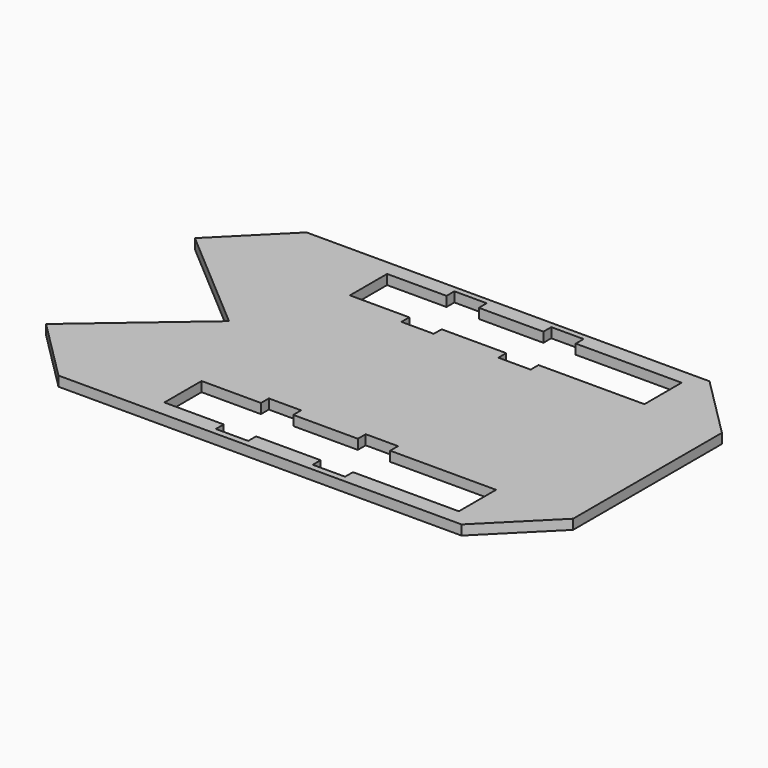
from build123d import *

# Parameters (mm, degrees)
F1_DEPTH = 3.175


# Not quite as in the source:
# - a length typed as a fraction of an inch, garbled in the dataset ("3 / 203.2 mm" for 3/8 in), is restored


with BuildPart() as f1:
    # F0 (on Top) → F1 (new body)
    with BuildSketch(Plane.XY):
        Polygon((84.4656275958, 81.8700266516), (-45.5343724042, 81.8700266516), (-65.5343724042, 61.8700266516), (-30.5343724042, 31.8700266516), (-65.5343724042, 1.8700266516), (-45.5343724042, -18.1299733484), (84.4656275958, -18.1299733484), (104.4656275958, 1.8700266516), (104.4656275958, 61.8700266516), align=None)
        Polygon((-15.5343724042, -12.9424554378), (-15.5343724042, 2.0575445622), (3.6249275958, 2.0575445622), (3.6249275958, 5.2325445622), (14.0516275958, 5.2325445622), (14.0516275958, 2.0575445622), (34.8796275958, 2.0575445622), (34.8796275958, 5.2325445622), (45.3063275958, 5.2325445622), (45.3063275958, 2.0575445622), (64.4656275958, 2.0575445622), (74.4656275958, 2.0575445622), (79.4656275958, 2.0575445622), (79.4656275958, -12.9424554378), (74.4656275958, -12.9424554378), (64.4656275958, -12.9424554378), (45.3063275958, -12.9424554378), (45.3063275958, -16.1174554378), (34.8796275958, -16.1174554378), (34.8796275958, -12.9424554378), (14.0516275958, -12.9424554378), (14.0516275958, -16.1174554378), (3.6249275958, -16.1174554378), (3.6249275958, -12.9424554378), align=None, mode=Mode.SUBTRACT)
        Polygon((-15.5343724042, 61.8700266516), (-15.5343724042, 76.8700266516), (3.6249275958, 76.8700266516), (3.6249275958, 80.0450266516), (14.0516275958, 80.0450266516), (14.0516275958, 76.8700266516), (34.8796275958, 76.8700266516), (34.8796275958, 80.0450266516), (45.3063275958, 80.0450266516), (45.3063275958, 76.8700266516), (64.4656275958, 76.8700266516), (74.4656275958, 76.8700266516), (79.4656275958, 76.8700266516), (79.4656275958, 61.8700266516), (74.4656275958, 61.8700266516), (64.4656275958, 61.8700266516), (45.3063275958, 61.8700266516), (45.3063275958, 58.6950266516), (34.8796275958, 58.6950266516), (34.8796275958, 61.8700266516), (14.0516275958, 61.8700266516), (14.0516275958, 58.6950266516), (3.6249275958, 58.6950266516), (3.6249275958, 61.8700266516), align=None, mode=Mode.SUBTRACT)
    extrude(amount=F1_DEPTH)


solid = f1.part
